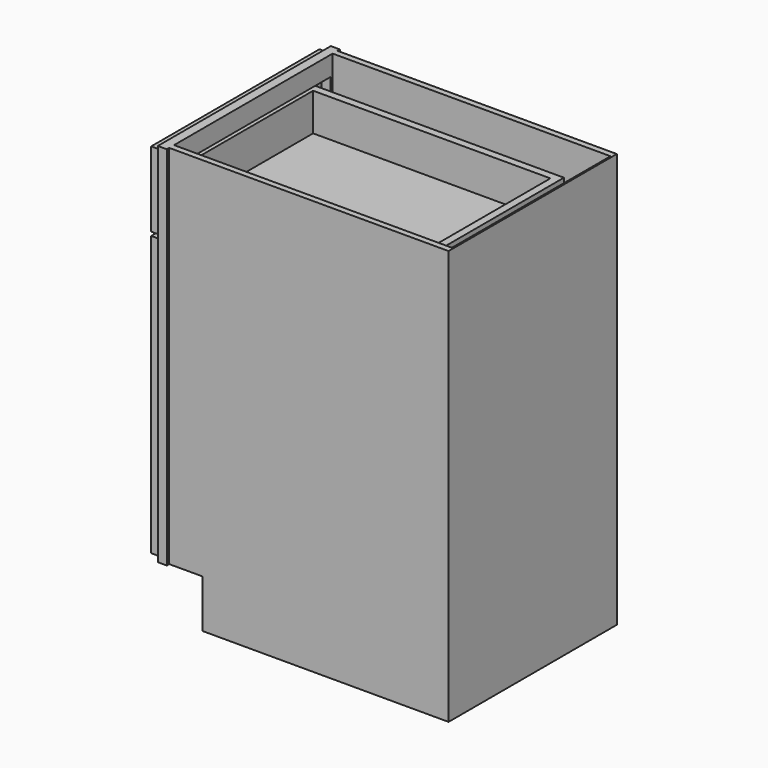
from build123d import *

# Parameters (mm, degrees)
F0_W          = 609.6
F0_H          = 876.3
F1_DEPTH      = 457.2
F2_W          = 88.9
F2_H          = 101.6
F3_DEPTH      = 457.201
F4_W          = 408.4819672131
F4_H          = 692.15
F5_DEPTH      = 19.05
F6_W          = 590.55
F6_H          = 6.35
F7_DEPTH      = 876.301
F8_W          = 587.375
F8_H          = 419.1
F9_DEPTH      = 733.425
F10_W         = 408.4819672131
F10_H         = 41.275
F11_DEPTH     = 19.05
F12_W         = 444.5
F12_H         = 590.5627
F12_W_2       = 330.2
F12_H_2       = 476.2627
F13_DEPTH     = 19.05
F14_W         = 6.35
F14_H         = 330.2
F15_DEPTH     = 476.2627
F16_SIZE      = 3.175
F17_W         = 444.5
F17_H         = 158.75
F17_W_2       = 330.2
F17_H_2       = 82.55
F18_DEPTH     = 19.05
F19_W         = 6.35
F19_H         = 330.2
F20_DEPTH     = 82.55
F21_SIZE      = 3.175
F22_W         = 504.825
F22_H         = 419.1
F23_DEPTH     = 101.6
F24_W         = 355.6
F24_H         = 95.25
F25_DEPTH     = 533.4
F26_T         = 15.875
F26_T3_DEPTH  = 37.249261314
F26_T5_DEPTH  = 37.249261314
F26_T7_DEPTH  = 37.249261314
F26_T9_DEPTH  = 37.249261314
F26_T11_DEPTH = 36.5125
F26_T13_DEPTH = 361.95
F26_T15_DEPTH = 114.3
F26_T17_DEPTH = 127
F26_T19_DEPTH = 387.35
F26_T21_DEPTH = 111.125
F26_T23_DEPTH = 36.5125


# Not quite as in the source:
# - a shell that OpenCascade refuses in one call is made with other operations: the cavity is built on its own and cut out


with BuildPart() as f1:
    # F0 (on Front) → F1 (new body)
    with BuildSketch(Plane.XZ):
        Rectangle(F0_W, F0_H)
    extrude(amount=-F1_DEPTH)

    # F2 (on face) → F3 (cut, through all)
    with BuildSketch(Plane.XZ):
        with Locations((-260.35, -387.35)):
            Rectangle(F2_W, F2_H)
    extrude(amount=-F3_DEPTH, mode=Mode.SUBTRACT)

    # F4 (on face) → F5 (cut)
    with BuildSketch(Plane(origin=(-304.8, 0, 0), x_dir=(0, -1, 0), z_dir=(-1, 0, 0))):
        with Locations((-228.6, 50.8)):
            Rectangle(F4_W, F4_H)
    extrude(amount=-F5_DEPTH, mode=Mode.SUBTRACT)

    # F6 (on face) → F7 (cut, through all)
    with BuildSketch(Plane.XY.offset(438.15)):
        with Locations((9.525, 454.025)):
            Rectangle(F6_W, F6_H)
        with Locations((9.525, 3.175)):
            Rectangle(F6_W, F6_H)
    extrude(amount=-F7_DEPTH, mode=Mode.SUBTRACT)

    # F8 (on face) → F9 (cut, through all)
    with BuildSketch(Plane.XY.offset(438.15)):
        with Locations((7.9375, 228.6)):
            Rectangle(F8_W, F8_H)
    extrude(amount=-F9_DEPTH, mode=Mode.SUBTRACT)

    # F10 (on face) → F11 (join, through all)
    with BuildSketch(Plane(origin=(-304.8, 0, 0), x_dir=(0, -1, 0), z_dir=(-1, 0, 0))):
        with Locations((-228.6, 265.1125)):
            Rectangle(F10_W, F10_H)
    extrude(amount=-F11_DEPTH)

    # F22 (on face) → F23 (cut)
    with BuildSketch(Plane(origin=(0, 0, -438.15), x_dir=(1, 0, 0), z_dir=(0, 0, -1))):
        with Locations((49.2125, -228.6)):
            Rectangle(F22_W, F22_H)
    extrude(amount=-F23_DEPTH, mode=Mode.SUBTRACT)


with BuildPart() as f13:
    # F12 (on face) → F13 (new body)
    with BuildSketch(Plane(origin=(-304.8, 0, 0), x_dir=(0, -1, 0), z_dir=(-1, 0, 0))):
        with Locations((-228.6, -33.33115)):
            Rectangle(F12_W, F12_H)
        with Locations((-228.6, -33.33115)):
            Rectangle(F12_W_2, F12_H_2, mode=Mode.SUBTRACT)
    extrude(amount=F13_DEPTH)

    # F14 (on face) → F15 (join, through all)
    with BuildSketch(Plane.XY.offset(-271.4625)):
        with Locations((-312.7375, 228.6)):
            Rectangle(F14_W, F14_H)
    extrude(amount=F15_DEPTH)

    # F16
    f16_edges = [f13.edges().sort_by_distance(p)[0] for p in [
        (-323.85, 393.7, -33.33115),
        (-323.85, 228.6, -271.4625),
        (-323.85, 63.5, -33.33115),
        (-323.85, 228.6, 204.8002),
    ]]
    chamfer(f16_edges, length=F16_SIZE)


with BuildPart() as f18:
    # F17 (on face) → F18 (new body)
    with BuildSketch(Plane(origin=(-304.8, 0, 0), x_dir=(0, -1, 0), z_dir=(-1, 0, 0))):
        with Locations((-228.6, 349.25)):
            Rectangle(F17_W, F17_H)
        with Locations((-228.6, 349.25)):
            Rectangle(F17_W_2, F17_H_2, mode=Mode.SUBTRACT)
    extrude(amount=F18_DEPTH)

    # F19 (on face) → F20 (join, through all)
    with BuildSketch(Plane.XY.offset(307.975)):
        with Locations((-312.7375, 228.6)):
            Rectangle(F19_W, F19_H)
    extrude(amount=F20_DEPTH)

    # F21
    f21_edges = [f18.edges().sort_by_distance(p)[0] for p in [
        (-323.85, 228.6, 307.975),
        (-323.85, 393.7, 349.25),
        (-323.85, 228.6, 390.525),
        (-323.85, 63.5, 349.25),
    ]]
    chamfer(f21_edges, length=F21_SIZE)

    # F24 (on face) → F25 (join)
    with BuildSketch(Plane.YZ.offset(-304.8)):
        with Locations((228.6, 339.725)):
            Rectangle(F24_W, F24_H)
    extrude(amount=F25_DEPTH)

    # F26: shell of thickness 15.875, made by hand


with BuildPart() as f26_core1:
    # F26_t2: copy of F18
    add(f18.part)

    # the walls: a layer under each face that stays
    f26_faces = [f26_core1.faces().sort_by_distance(p)[0] for p in [
        (-323.85, 376.7666666667, 296.3333333333),
        (-322.2625, 228.6, 306.3875),
        (-322.2625, 61.9125, 349.25),
        (-322.2625, 395.2875, 349.25),
        (-322.2625, 228.6, 392.1125),
        (-314.325, 228.6, 428.625),
        (-314.325, 450.85, 349.25),
        (-314.325, 228.6, 269.875),
        (-314.325, 6.35, 349.25),
        (-318.29375, 228.6, 307.975),
        (-318.29375, 63.5, 349.25),
        (-318.29375, 393.7, 349.25),
        (-318.29375, 228.6, 390.525),
        (-304.8, 376.7666666667, 402.1666666667),
        (-315.9125, 228.6, 349.25),
        (-38.1, 406.4, 339.725),
        (-38.1, 228.6, 292.1),
        (-38.1, 50.8, 339.725),
        (-307.18125, 63.5, 349.25),
        (-307.18125, 228.6, 390.525),
        (-307.18125, 393.7, 349.25),
        (-304.8, 228.6, 347.6625),
        (228.6, 228.6, 339.725),
        (-307.18125, 228.6, 307.975),
        (-309.5625, 228.6, 349.25),
    ]]
    thicken(f26_faces, amount=-F26_T, mode=Mode.SUBTRACT)

    # F26_s4 → F26_t3 (cut)
    with BuildSketch(Plane(origin=(4.5928978099, 4.5928978099, 4.5928978099), x_dir=(-0.7071067812, 0.7071067812, 0), z_dir=(0.5773502692, 0.5773502692, 0.5773502692))):
        Polygon((271.8908726623, 356.5892701441), (263.7152476623, 342.7036353262), (255.7777476623, 347.2863530879), (255.7777476623, 356.4517886113), align=None)
    extrude(amount=F26_T3_DEPTH, mode=Mode.SUBTRACT)

    # F26_s6 → F26_t5 (cut)
    with BuildSketch(Plane(origin=(-147.8071021901, 147.8071021901, -147.8071021901), x_dir=(0.7071067812, 0.7071067812, 0), z_dir=(0.5773502692, -0.5773502692, 0.5773502692))):
        Polygon((51.3983476961, 543.2403885442), (59.5739726961, 529.3547537263), (67.5114726961, 533.937471488), (67.5114726961, 543.1029070113), align=None)
    extrude(amount=F26_T5_DEPTH, mode=Mode.SUBTRACT)

    # F26_s8 → F26_t7 (cut)
    with BuildSketch(Plane(origin=(-228.2404355234, -228.2404355234, 228.2404355234), x_dir=(-0.7071067812, 0.7071067812, 0), z_dir=(0.5773502692, 0.5773502692, -0.5773502692))):
        Polygon((271.8908726623, 213.7335916339), (255.7777476623, 213.8710731668), (255.7777476623, 223.0365086901), (263.7152476623, 227.6192264518), align=None)
    extrude(amount=F26_T7_DEPTH, mode=Mode.SUBTRACT)

    # F26_s10 → F26_t9 (cut)
    with BuildSketch(Plane(origin=(-380.6404355234, 380.6404355234, 380.6404355234), x_dir=(0.7071067812, 0.7071067812, 0), z_dir=(0.5773502692, -0.5773502692, -0.5773502692))):
        Polygon((51.3983476961, 27.0824732338), (67.5114726961, 27.2199547667), (67.5114726961, 36.3853902901), (59.5739726961, 40.9681080518), align=None)
    extrude(amount=F26_T9_DEPTH, mode=Mode.SUBTRACT)

    # F26_s12 → F26_t11 (cut)
    with BuildSketch(Plane.YZ.offset(-336.55)):
        Polygon((393.54125, 308.13375), (393.7, 292.1), (409.575, 292.1), (409.575, 307.975), align=None)
        Polygon((63.65875, 308.13375), (63.5, 292.1), (47.625, 292.1), (47.625, 307.975), align=None)
        Polygon((63.65875, 390.36625), (47.625, 390.525), (47.625, 406.4), (63.5, 406.4), align=None)
        Polygon((393.54125, 390.36625), (409.575, 390.525), (409.575, 406.4), (393.7, 406.4), align=None)
    extrude(amount=F26_T11_DEPTH, mode=Mode.SUBTRACT)

    # F26_s14 → F26_t13 (cut)
    with BuildSketch(Plane.XZ.offset(-409.575)):
        Polygon((-316.07125, 308.13375), (-315.9125, 292.1), (-300.0375, 292.1), (-300.0375, 307.975), align=None)
        Polygon((-316.07125, 390.36625), (-315.9125, 406.4), (-300.0375, 406.4), (-300.0375, 390.525), align=None)
        Polygon((-309.40375, 390.36625), (-309.5625, 406.4), (-325.4375, 406.4), (-325.4375, 390.525), align=None)
        Polygon((-304.95875, 308.13375), (-288.925, 307.975), (-288.925, 292.1), (-304.8, 292.1), align=None)
        Polygon((-309.40375, 308.13375), (-309.5625, 292.1), (-325.4375, 292.1), (-325.4375, 307.975), align=None)
    extrude(amount=F26_T13_DEPTH, mode=Mode.SUBTRACT)

    # F26_s16 → F26_t15 (cut)
    with BuildSketch(Plane.XY.offset(292.1)):
        Polygon((-316.07125, 63.65875), (-315.9125, 47.625), (-300.0375, 47.625), (-300.0375, 63.5), align=None)
        Polygon((-316.07125, 393.54125), (-315.9125, 409.575), (-300.0375, 409.575), (-300.0375, 393.7), align=None)
        Polygon((-309.40375, 63.65875), (-309.5625, 47.625), (-325.4375, 47.625), (-325.4375, 63.5), align=None)
        Polygon((-309.40375, 393.54125), (-309.5625, 409.575), (-325.4375, 409.575), (-325.4375, 393.7), align=None)
    extrude(amount=F26_T15_DEPTH, mode=Mode.SUBTRACT)

    # F26_s18 → F26_t17 (cut)
    with BuildSketch(Plane.XY.offset(276.225)):
        Polygon((-304.64125, 406.55875), (-320.675, 406.4), (-320.675, 390.525), (-304.8, 390.525), align=None)
        Polygon((-304.64125, 50.64125), (-320.675, 50.8), (-320.675, 66.675), (-304.8, 66.675), align=None)
    extrude(amount=F26_T17_DEPTH, mode=Mode.SUBTRACT)

    # F26_s20 → F26_t19 (cut)
    with BuildSketch(Plane.XZ.offset(-422.275)):
        Polygon((-304.64125, 291.94125), (-320.675, 292.1), (-320.675, 307.975), (-304.8, 307.975), align=None)
    extrude(amount=F26_T19_DEPTH, mode=Mode.SUBTRACT)

    # F26_s22 → F26_t21 (cut)
    with BuildSketch(Plane.XY.offset(292.1)):
        Polygon((-304.95875, 63.65875), (-304.8, 47.625), (-288.925, 47.625), (-288.925, 63.5), align=None)
        Polygon((-304.95875, 393.54125), (-304.8, 409.575), (-288.925, 409.575), (-288.925, 393.7), align=None)
    extrude(amount=F26_T21_DEPTH, mode=Mode.SUBTRACT)

    # F26_s24 → F26_t23 (cut)
    with BuildSketch(Plane.YZ.offset(-325.4375)):
        Polygon((63.65875, 308.13375), (47.625, 307.975), (47.625, 292.1), (63.5, 292.1), align=None)
        Polygon((63.65875, 390.36625), (47.625, 390.525), (47.625, 406.4), (63.5, 406.4), align=None)
        Polygon((393.54125, 390.36625), (393.7, 406.4), (409.575, 406.4), (409.575, 390.525), align=None)
        Polygon((393.54125, 308.13375), (409.575, 307.975), (409.575, 292.1), (393.7, 292.1), align=None)
    extrude(amount=F26_T23_DEPTH, mode=Mode.SUBTRACT)


with BuildPart() as f18_1:
    add(f18.part)

    # what is left inside the walls is the cavity
    f26_cavity = [f26_core1.part.solids().sort_by_distance(p)[0] for p in [
        (45.508333, 228.6, 308.13375),
    ]]
    add(f26_cavity, mode=Mode.SUBTRACT)


solid = Compound([f1.part, f13.part, f18_1.part])
